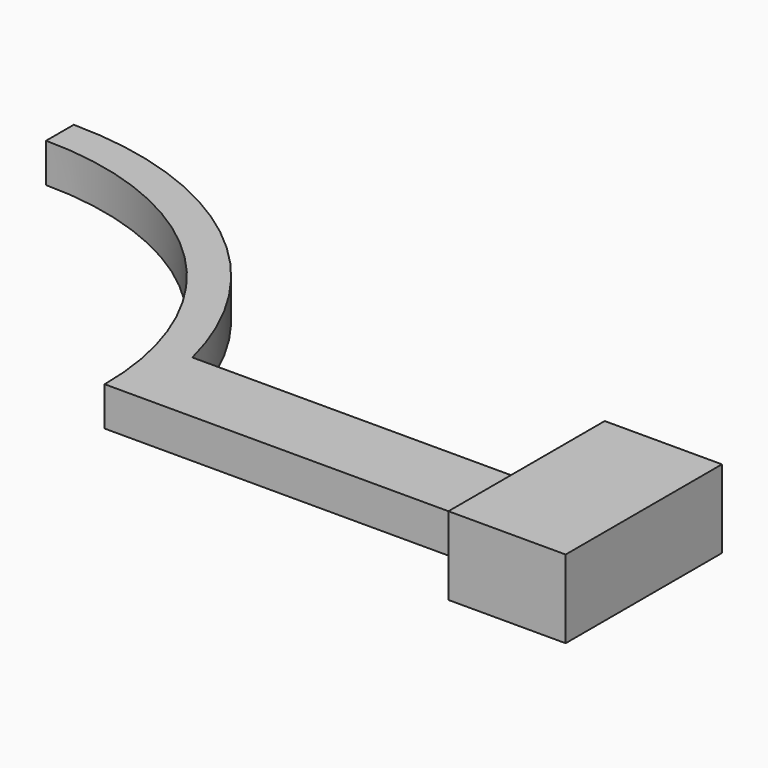
from build123d import *

# Parameters (mm, degrees)
F0_W     = 7.62
F0_H     = 12.7
F1_DEPTH = 5.08
F2_W     = 5.08
F2_H     = 2.54
F3_DEPTH = 25.4
F5_DEPTH = 2.54


# Not quite as in the source:
# - a feature names something its author has since deleted; it is built from what else it names


with BuildPart() as f1:
    # F0 (on Top) → F1 (new body)
    with BuildSketch(Plane.XY):
        with Locations((-65.9446567297, 13.238232059)):
            Rectangle(F0_W, F0_H)
    extrude(amount=F1_DEPTH)

    # F2 (on face) → F3 (join)
    with BuildSketch(Plane(origin=(-69.7546567297, 0, 0), x_dir=(0, -1, 0), z_dir=(-1, 0, 0))):
        with Locations((-13.238232059, 1.27)):
            Rectangle(F2_W, F2_H)
    extrude(amount=F3_DEPTH)

    # F4 (on face) → F5 (join)
    with BuildSketch(Plane(origin=(0, 0, 0), x_dir=(1, 0, 0), z_dir=(0, 0, -1))):
        with BuildLine():
            Line((-93.5208049366, -15.778232059), (-95.1546567297, -15.778232059))
            Line((-95.1546567297, -15.778232059), (-95.1546567297, -10.698232059))
            ThreePointArc((-95.1546567297, -10.698232059), (-100.7342725481, -24.1686162406), (-114.2046567297, -29.748232059))
            Line((-114.2046567297, -29.748232059), (-114.2046567297, -31.9967795447))
            ThreePointArc((-114.2046567297, -31.9967795447), (-101.0625202258, -27.4586727786), (-93.5208049366, -15.778232059))
        make_face()
    extrude(amount=-F5_DEPTH)


solid = f1.part
